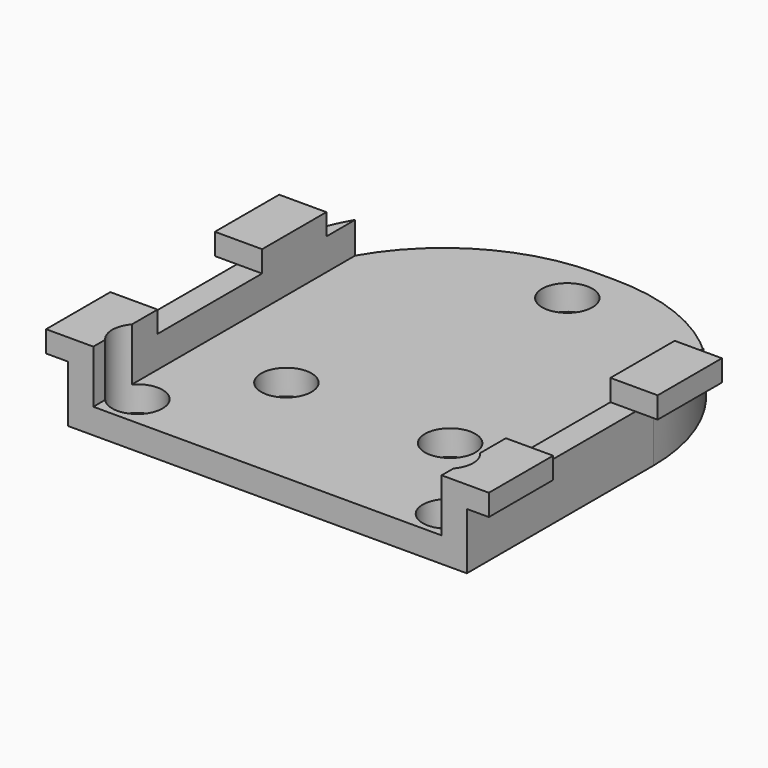
from build123d import *

# Parameters (mm, degrees)
F0_W         = 63.3
F0_H         = 67
F1_DEPTH     = 4
F3_W         = 4
F3_H         = 67
F4_DEPTH     = 5
F6_W         = 7.5
F6_H         = 12.75
F7_DEPTH     = 3.4
F2_R         = 4
F9_DEPTH     = 25
F8_R         = 4
F10_DEPTH    = 25
F11_T1_DEPTH = 84
F12_T1_DEPTH = 84


# Not quite as in the source:
# - a fillet or chamfer that OpenCascade refuses, or shapes differently, is made with other operations: its cross-section is extruded or revolved along the edge and cut away or added


with BuildPart() as f1:
    # F0 (on Top) → F1 (new body)
    with BuildSketch(Plane.XY):
        Rectangle(F0_W, F0_H)
    extrude(amount=F1_DEPTH)

    # F3 (on face) → F4 (join)
    with BuildSketch(Plane.XY.offset(4)):
        with Locations((-29.65, 0)):
            Rectangle(F3_W, F3_H)
        with Locations((29.65, 0)):
            Rectangle(F3_W, F3_H)
    extrude(amount=F4_DEPTH)

    # F6 (on face) → F7 (join)
    with BuildSketch(Plane.XY.offset(9)):
        with Locations((-31.4, 6.375)):
            Rectangle(F6_W, F6_H)
        with Locations((-31.4, -27.125)):
            Rectangle(F6_W, F6_H)
        with Locations((31.4, -27.125)):
            Rectangle(F6_W, F6_H)
        with Locations((31.4, 6.375)):
            Rectangle(F6_W, F6_H)
    extrude(amount=F7_DEPTH)

    # F2 (on Top) → F9 (cut)
    with BuildSketch(Plane.XY):
        with Locations((-24.65, -28.5)):
            Circle(F2_R)
        with Locations((24.65, -28.5)):
            Circle(F2_R)
    extrude(amount=F9_DEPTH, mode=Mode.SUBTRACT)

    # F8 (on Top) → F10 (cut)
    with BuildSketch(Plane.XY):
        with Locations((0, 26)):
            Circle(F8_R)
        with Locations((-13, -13.5)):
            Circle(F8_R)
        with Locations((13, -13.5)):
            Circle(F8_R)
    extrude(amount=F10_DEPTH, mode=Mode.SUBTRACT)

    # F11: fillet of radius 30 on 1 edges, made by hand

    # F11_s2 → F11_t1 (cut)
    with BuildSketch(Plane.XY.offset(-75)):
        with BuildLine():
            ThreePointArc((-1.65, 33.5), (-22.8632034356, 24.7132034356), (-31.65, 3.5))
            Line((-31.65, 3.5), (-31.65, 33.5))
            Line((-31.65, 33.5), (-1.65, 33.5))
        make_face()
    extrude(amount=F11_T1_DEPTH, mode=Mode.SUBTRACT)

    # F12: fillet of radius 30 on 1 edges, made by hand

    # F12_s2 → F12_t1 (cut)
    with BuildSketch(Plane.XY.offset(-75)):
        with BuildLine():
            ThreePointArc((31.65, 3.5), (22.8632034356, 24.7132034356), (1.65, 33.5))
            Line((1.65, 33.5), (31.65, 33.5))
            Line((31.65, 33.5), (31.65, 3.5))
        make_face()
    extrude(amount=F12_T1_DEPTH, mode=Mode.SUBTRACT)


solid = f1.part
